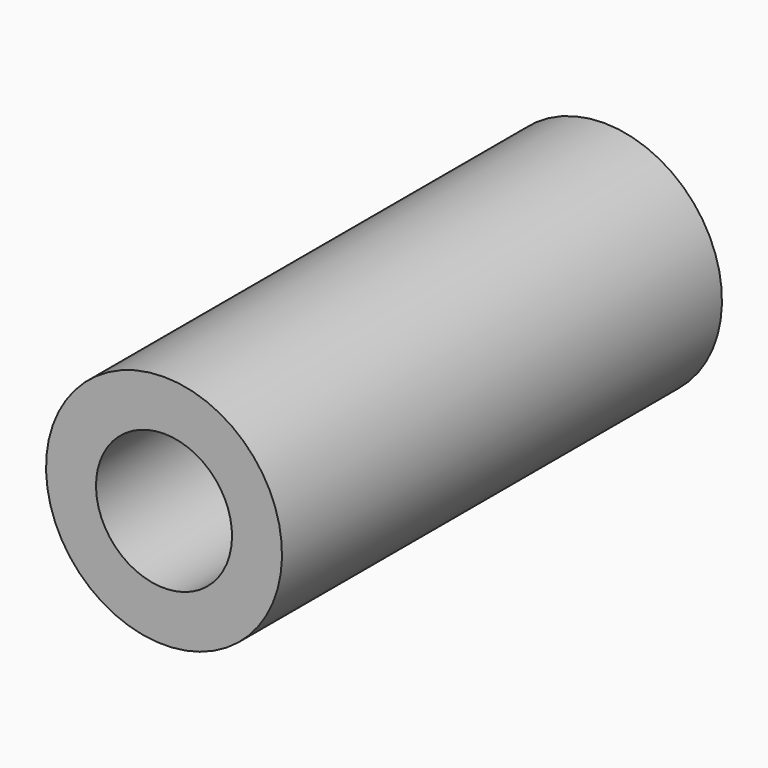
from build123d import *

# Parameters (mm, degrees)
F2_SIZE = 0.09999


# Not quite as in the source:
# - a fillet or chamfer is up to 0.001 mm smaller than in the source, because OpenCascade refuses the exact size


with BuildPart() as f1:
    # F0 (on Right) → F1 (revolve)
    with BuildSketch(Plane.YZ):
        Polygon((6.425, 3.3), (6.925, 2.8), (6.925, 3.3), align=None)
        with BuildLine():
            ThreePointArc((7.5617104388, 2.8), (8.3591026496, 4.0638625595), (9.425, 5.1112620751))
            Line((9.425, 5.1112620751), (9.425, 5.9))
            Line((9.425, 5.9), (-18.075, 5.9))
            Line((-18.075, 5.9), (-18.075, 3.4))
            Line((-18.075, 3.4), (-7.075, 3.4))
            Line((-7.075, 3.4), (-7.075, 3.3))
            Line((-7.075, 3.3), (-6.425, 3.3))
            Line((-6.425, 3.3), (6.425, 3.3))
            Line((6.425, 3.3), (6.925, 3.3))
            Line((6.925, 3.3), (6.925, 2.8))
            Line((6.925, 2.8), (7.5617104388, 2.8))
        make_face()
    revolve(axis=Axis((0, 1.2040399015, 0), (0, 1, 0)))

    # F2 (size 0.1 in the source; OpenCascade refuses exactly that, so slightly less here)
    f2_edges = [f1.edges().sort_by_distance(p)[0] for p in [
        (0, -7.075, -3.4),
    ]]
    chamfer(f2_edges, length=F2_SIZE)


solid = f1.part
